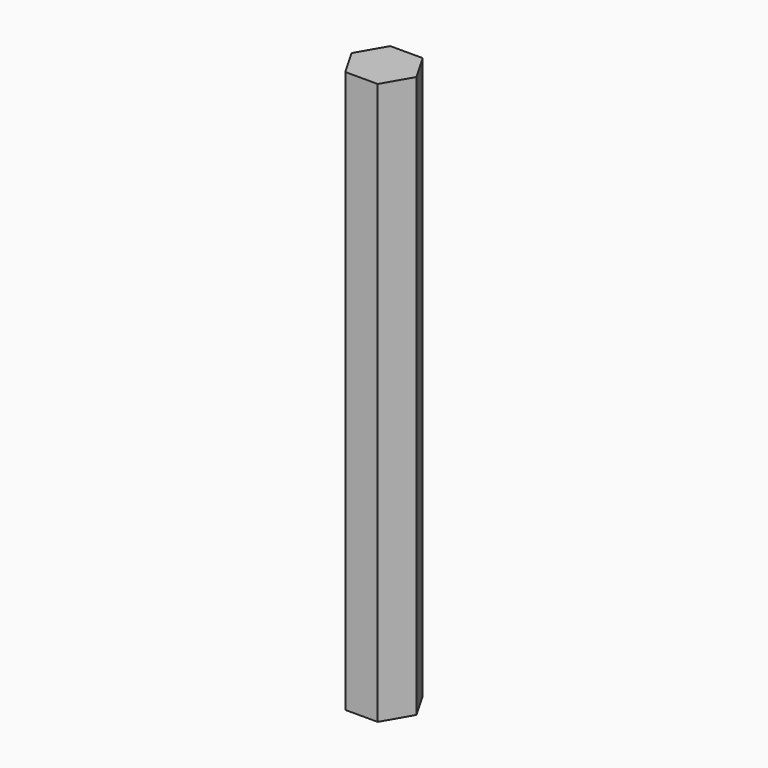
from build123d import *

# Parameters (mm, degrees)
F2_DEPTH = 127


# Not quite as in the source:
# - a variable given as a bare number and used for a length is read in inches; the dataset says mm whatever the document's units were


with BuildPart() as f2:
    # F1 (on Top) → F2 (new body)
    with BuildSketch(Plane.XY):
        Polygon((3.6661742094, 6.35), (-3.6661742094, 6.35), (-7.3323484187, 0), (-3.6661742094, -6.35), (3.6661742094, -6.35), (7.3323484187, 0), align=None)
    extrude(amount=F2_DEPTH)


solid = f2.part
